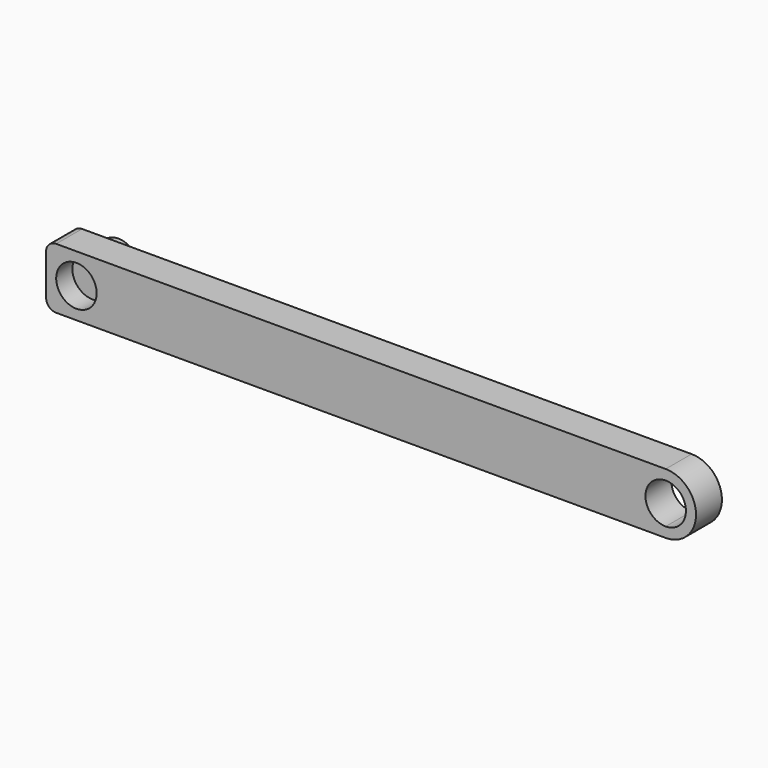
from build123d import *

# Parameters (mm, degrees)
F1_DEPTH = 8
F2_R     = 2.5
F3_R     = 5
F4_DEPTH = 5
F5_R     = 5
F6_DEPTH = 5


# Not quite as in the source:
# - a feature names something its author has since deleted; it is built from what else it names


with BuildPart() as f1:
    # F0 (on Front) → F1 (new body)
    with BuildSketch(Plane.XZ):
        with BuildLine():
            ThreePointArc((0, -7.5), (-7.5, 0), (0, 7.5))
            Line((0, 7.5), (-153.126, 7.5))
            Line((-153.126, 7.5), (-153.126, -7.5))
            Line((-153.126, -7.5), (0, -7.5))
        make_face()
        with BuildLine():
            Line((0, 5), (0, 7.5))
            ThreePointArc((0, 7.5), (-7.5, 0), (0, -7.5))
            Line((0, -7.5), (0, -5))
            ThreePointArc((0, -5), (-5, 0), (0, 5))
        make_face()
        with BuildLine():
            ThreePointArc((0, -7.5), (5.3033008589, -5.3033008589), (7.5, 0))
            ThreePointArc((7.5, 0), (5.3033008589, 5.3033008589), (0, 7.5))
            Line((0, 7.5), (0, 5))
            ThreePointArc((0, 5), (3.5355339059, 3.5355339059), (5, 0))
            ThreePointArc((5, 0), (3.5355339059, -3.5355339059), (0, -5))
            Line((0, -5), (0, -7.5))
        make_face()
    extrude(amount=F1_DEPTH)

    # F2
    f2_edges = [f1.edges().sort_by_distance(p)[0] for p in [
        (-153.126, -4, 7.5),
        (-153.126, -4, -7.5),
    ]]
    fillet(f2_edges, radius=F2_R)

    # F3 (on face) → F4 (join)
    with BuildSketch(Plane(origin=(0, 0, 0), x_dir=(-1, 0, 0), z_dir=(0, 1, 0))):
        with Locations((145.626, 0)):
            Circle(F3_R)
    extrude(amount=F4_DEPTH)

    # F5 (on face) → F6 (cut)
    with BuildSketch(Plane.XZ.offset(8)):
        with Locations((-145.626, 0)):
            Circle(F5_R)
    extrude(amount=-F6_DEPTH, mode=Mode.SUBTRACT)


solid = f1.part
